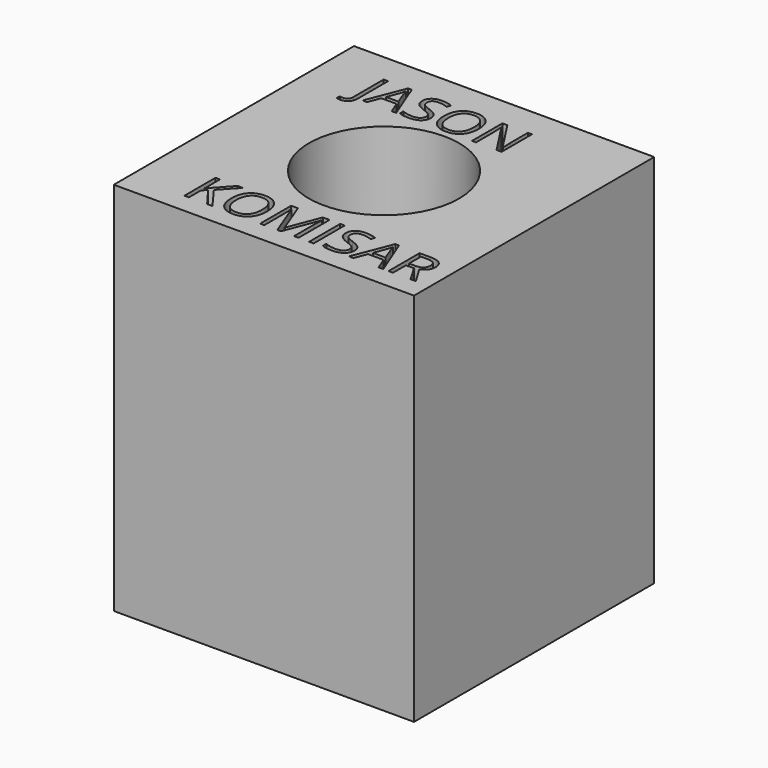
from build123d import *

# Parameters (mm, degrees)
F0_W           = 101.6
F0_H           = 101.6
F1_DEPTH       = 101.6
F2_R           = 25.4
F3_DEPTH       = 101.6
F4_DEPTH       = 25.4
F5_TEXT_SIZE   = 17.9878591249
F5_TEXT_SIZE_2 = 18.387595709
F6_DEPTH       = 152.4


# Not quite as in the source:
# - Text() gives the source's letters only with a copy of the font that has no kerning and outlines rounded to 1/6400 em; it was checked with that copy


with BuildPart() as f1:
    # F0 (on Top) → F1 (new body)
    with BuildSketch(Plane.XY):
        Rectangle(F0_W, F0_H)
    extrude(amount=F1_DEPTH)

    # F2 (on face) → F3 (cut)
    with BuildSketch(Plane.XY.offset(101.6)):
        Circle(F2_R)
    extrude(amount=-F3_DEPTH, mode=Mode.SUBTRACT)

    # F4 (add): a face of the model
    f4_faces = [f1.faces().sort_by_distance(p)[0] for p in [
        (49.3631590206, 0, 101.6),
    ]]
    extrude(f4_faces, amount=F4_DEPTH)

    # F5 (on face) → F6 (cut)
    with BuildSketch(Plane.XY.offset(127)):
        with Locations((-34.3927890062, 27.9171578586)):
            Text('JASON', F5_TEXT_SIZE, font='Open Sans', text_align=(TextAlign.LEFT, TextAlign.BOTTOM))
        with Locations((-34.1049842536, -44.0342836082)):
            Text('KOMISAR', F5_TEXT_SIZE_2, font='Open Sans', text_align=(TextAlign.LEFT, TextAlign.BOTTOM))
    extrude(amount=-F6_DEPTH, mode=Mode.SUBTRACT)


solid = f1.part
